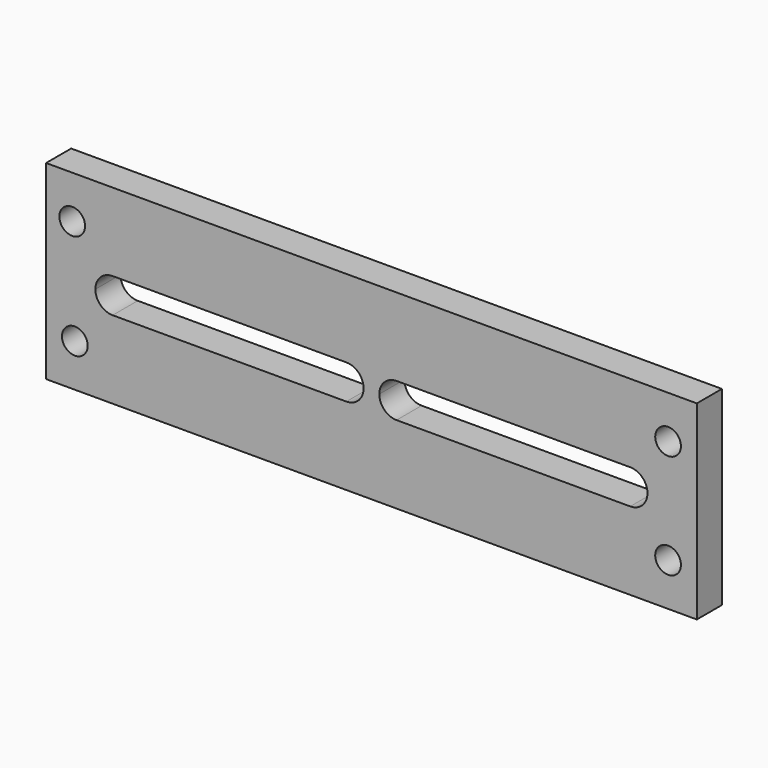
from build123d import *

# Parameters (mm, degrees)
F0_W     = 124.5
F0_H     = 36.4
F0_R     = 2.46
F0_W_2   = 51.32
F0_H_2   = 6.6
F0_W_3   = 51.308
F1_DEPTH = 6
F2_R     = 3.3
F3_R     = 3.29999
F4_R     = 3.3
F5_R     = 3.29999
F6_R     = 3.3
F7_R     = 3.29999
F8_R     = 3.3
F9_R     = 3.29999


# Not quite as in the source:
# - a fillet or chamfer is up to 0.001 mm smaller than in the source, because OpenCascade refuses the exact size


with BuildPart() as f1:
    # F0 (on Front) → F1 (new body)
    with BuildSketch(Plane.XZ):
        Rectangle(F0_W, F0_H)
        with Locations((-56.75, -10)):
            Circle(F0_R, mode=Mode.SUBTRACT)
        with Locations((-27.16, 0)):
            Rectangle(F0_W_2, F0_H_2, mode=Mode.SUBTRACT)
        with Locations((56.75, -10)):
            Circle(F0_R, mode=Mode.SUBTRACT)
        with Locations((27.154, 0)):
            Rectangle(F0_W_3, F0_H_2, mode=Mode.SUBTRACT)
        with Locations((-57.25, 10)):
            Circle(F0_R, mode=Mode.SUBTRACT)
        with Locations((56.75, 10)):
            Circle(F0_R, mode=Mode.SUBTRACT)
    extrude(amount=F1_DEPTH)

    # F2
    f2_edges = [f1.edges().sort_by_distance(p)[0] for p in [
        (-52.82, -3, -3.3),
    ]]
    fillet(f2_edges, radius=F2_R)

    # F3 (radius 3.3 in the source; OpenCascade refuses exactly that, so slightly less here)
    f3_edges = [f1.edges().sort_by_distance(p)[0] for p in [
        (-52.82, -3, 3.3),
    ]]
    fillet(f3_edges, radius=F3_R)

    # F4
    f4_edges = [f1.edges().sort_by_distance(p)[0] for p in [
        (-1.5, -3, 3.3),
    ]]
    fillet(f4_edges, radius=F4_R)

    # F5 (radius 3.3 in the source; OpenCascade refuses exactly that, so slightly less here)
    f5_edges = [f1.edges().sort_by_distance(p)[0] for p in [
        (-1.5, -3, -3.3),
    ]]
    fillet(f5_edges, radius=F5_R)

    # F6
    f6_edges = [f1.edges().sort_by_distance(p)[0] for p in [
        (1.5, -3, 3.3),
    ]]
    fillet(f6_edges, radius=F6_R)

    # F7 (radius 3.3 in the source; OpenCascade refuses exactly that, so slightly less here)
    f7_edges = [f1.edges().sort_by_distance(p)[0] for p in [
        (1.5, -3, -3.3),
    ]]
    fillet(f7_edges, radius=F7_R)

    # F8
    f8_edges = [f1.edges().sort_by_distance(p)[0] for p in [
        (52.808, -3, 3.3),
    ]]
    fillet(f8_edges, radius=F8_R)

    # F9 (radius 3.3 in the source; OpenCascade refuses exactly that, so slightly less here)
    f9_edges = [f1.edges().sort_by_distance(p)[0] for p in [
        (52.808, -3, -3.3),
    ]]
    fillet(f9_edges, radius=F9_R)


solid = f1.part
